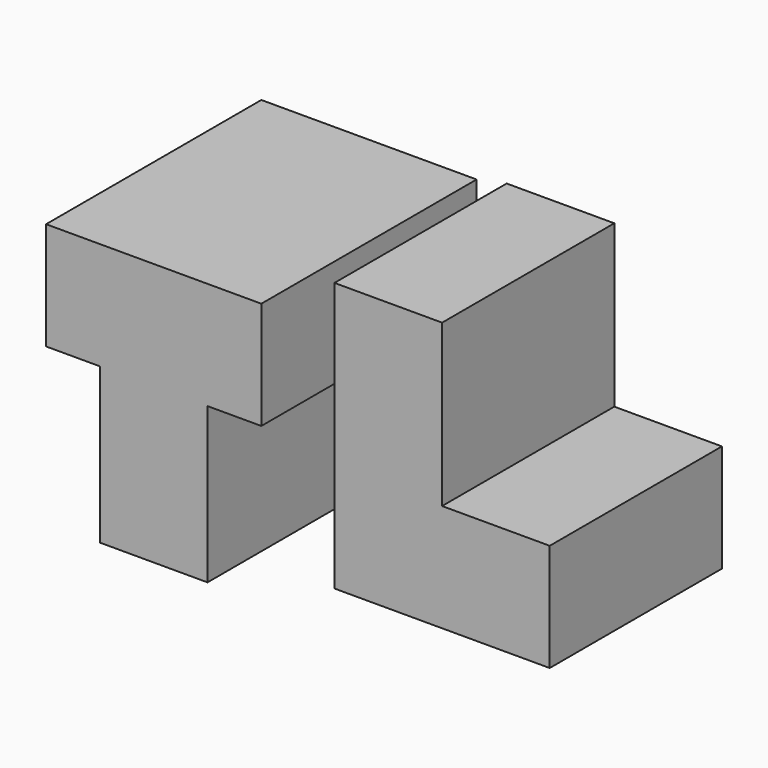
from build123d import *

# Parameters (mm, degrees)
F1_DEPTH = 25.4
F3_DEPTH = 31.75


# Not quite as in the source:
# - a length typed as a fraction of an inch, garbled in the dataset ("3 / 203.2 mm" for 3/8 in), is restored


with BuildPart() as f1:
    # F0 (on Front) → F1 (new body)
    with BuildSketch(Plane.XZ):
        Polygon((12.7, 31.75), (0, 31.75), (0, 0), (25.4, 0), (25.4, 12.7), (12.7, 12.7), align=None)
    extrude(amount=F1_DEPTH)


with BuildPart() as f3:
    # F2 (on Front) → F3 (new body)
    with BuildSketch(Plane.XZ):
        Polygon((-22.599989511, 0), (-9.899989511, 0), (-9.899989511, 18.3144848176), (-3.549989511, 18.3144848176), (-3.549989511, 31.0144848176), (-28.949989511, 31.0144848176), (-28.949989511, 18.3144848176), (-22.599989511, 18.3144848176), align=None)
    extrude(amount=F3_DEPTH)


solid = Compound([f1.part, f3.part])
